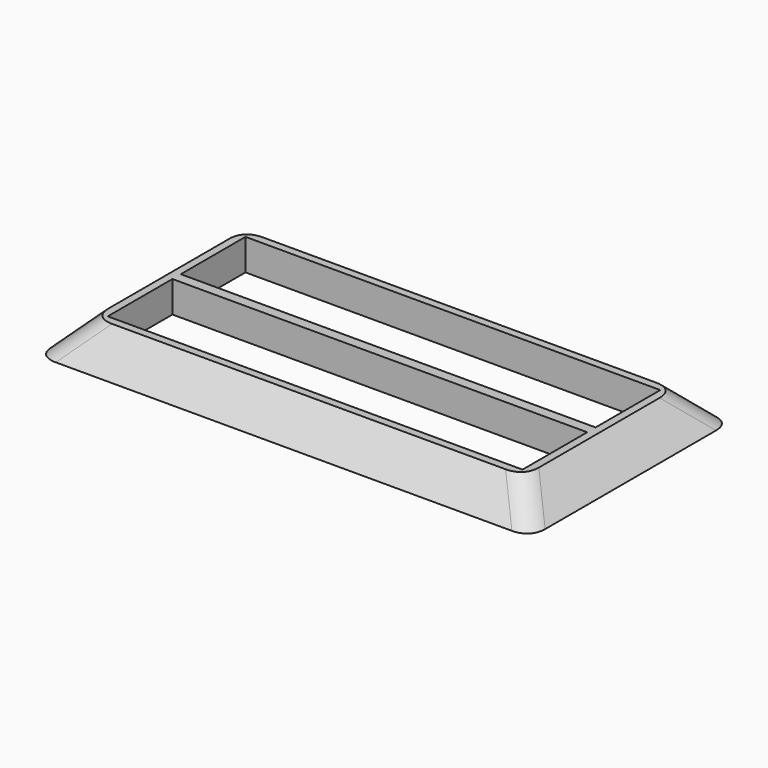
from build123d import *

# Parameters (mm, degrees)
F0_W        = 18.9
F0_H        = 9.6
F0_W_2      = 15.9
F0_H_2      = 3.1
F1_DEPTH    = 1.2
F2_SIZE     = 1.19999
F3_T1_DEPTH = 4.9651949945
F3_T3_DEPTH = 4.9651949945
F3_T5_DEPTH = 4.9651949945
F3_T7_DEPTH = 4.9651949945


# Not quite as in the source:
# - a fillet or chamfer that OpenCascade refuses, or shapes differently, is made with other operations: its cross-section is extruded or revolved along the edge and cut away or added
# - a fillet or chamfer is up to 0.001 mm smaller than in the source, because OpenCascade refuses the exact size


with BuildPart() as f1:
    # F0 (on Top) → F1 (new body)
    with BuildSketch(Plane.XY):
        Rectangle(F0_W, F0_H)
        with Locations((0, -1.75)):
            Rectangle(F0_W_2, F0_H_2, mode=Mode.SUBTRACT)
        with Locations((0, 1.75)):
            Rectangle(F0_W_2, F0_H_2, mode=Mode.SUBTRACT)
    extrude(amount=F1_DEPTH)

    # F2 (size 1.2 in the source; OpenCascade refuses exactly that, so slightly less here)
    f2_edges = [f1.edges().sort_by_distance(p)[0] for p in [
        (0, -4.8, 1.2),
        (-9.45, 0, 1.2),
        (9.45, 0, 1.2),
        (0, 4.8, 1.2),
    ]]
    chamfer(f2_edges, length=F2_SIZE)

    # F3: fillet of radius 1 on 4 edges, made by hand

    # F3_s2 → F3_t1 (cut)
    with BuildSketch(Plane(origin=(-5.58333, -5.58333, -5.58333), x_dir=(-0.7071067812, 0.7071067812, 0), z_dir=(0.5773502692, 0.5773502692, 0.5773502692))):
        with BuildLine():
            ThreePointArc((3.7880465325, 5.5288711695), (3.2880465325, 5.6628457657), (2.7880465325, 5.5288711695))
            Line((2.7880465325, 5.5288711695), (3.2880465325, 5.8175463041))
            Line((3.2880465325, 5.8175463041), (3.7880465325, 5.5288711695))
        make_face()
    extrude(amount=F3_T1_DEPTH, mode=Mode.SUBTRACT)

    # F3_s4 → F3_t3 (cut)
    with BuildSketch(Plane(origin=(5.58333, -5.58333, -5.58333), x_dir=(-0.7071067812, -0.7071067812, 0), z_dir=(-0.5773502692, 0.5773502692, 0.5773502692))):
        with BuildLine():
            ThreePointArc((-3.7880465325, 5.5288711695), (-3.2880465325, 5.6628457657), (-2.7880465325, 5.5288711695))
            Line((-2.7880465325, 5.5288711695), (-3.2880465325, 5.8175463041))
            Line((-3.2880465325, 5.8175463041), (-3.7880465325, 5.5288711695))
        make_face()
    extrude(amount=F3_T3_DEPTH, mode=Mode.SUBTRACT)

    # F3_s6 → F3_t5 (cut)
    with BuildSketch(Plane(origin=(5.58333, 5.58333, -5.58333), x_dir=(0.7071067812, -0.7071067812, 0), z_dir=(-0.5773502692, -0.5773502692, 0.5773502692))):
        with BuildLine():
            ThreePointArc((2.7880465325, 5.5288711695), (3.2880465325, 5.6628457657), (3.7880465325, 5.5288711695))
            Line((3.7880465325, 5.5288711695), (3.2880465325, 5.8175463041))
            Line((3.2880465325, 5.8175463041), (2.7880465325, 5.5288711695))
        make_face()
    extrude(amount=F3_T5_DEPTH, mode=Mode.SUBTRACT)

    # F3_s8 → F3_t7 (cut)
    with BuildSketch(Plane(origin=(-5.58333, 5.58333, -5.58333), x_dir=(0.7071067812, 0.7071067812, 0), z_dir=(0.5773502692, -0.5773502692, 0.5773502692))):
        with BuildLine():
            ThreePointArc((-2.7880465325, 5.5288711695), (-3.2880465325, 5.6628457657), (-3.7880465325, 5.5288711695))
            Line((-3.7880465325, 5.5288711695), (-3.2880465325, 5.8175463041))
            Line((-3.2880465325, 5.8175463041), (-2.7880465325, 5.5288711695))
        make_face()
    extrude(amount=F3_T7_DEPTH, mode=Mode.SUBTRACT)


solid = f1.part
